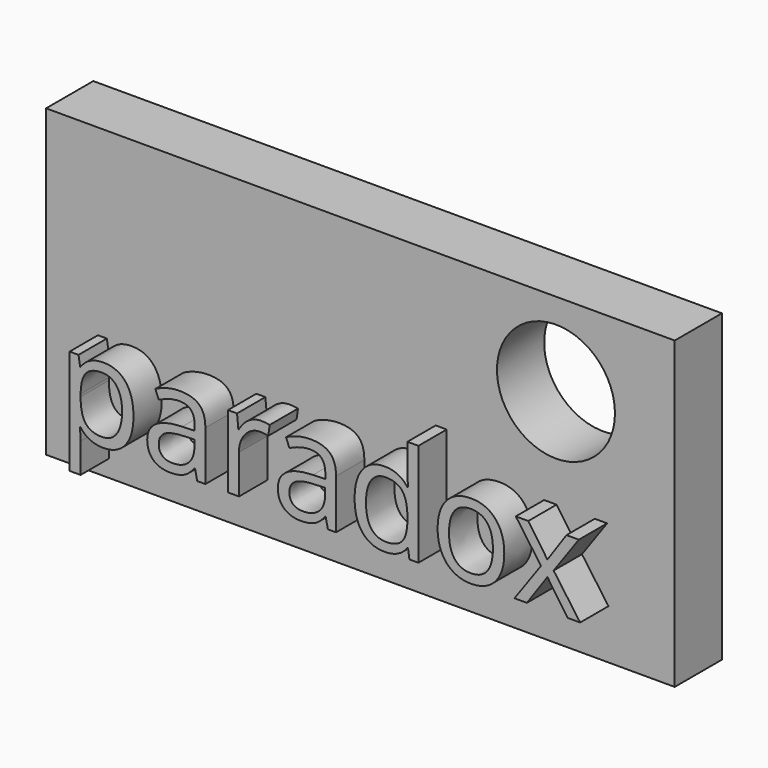
from build123d import *

# Parameters (mm, degrees)
F0_W         = 53.2775521278
F0_H         = 25.8456766605
F1_DEPTH     = 5
F2_TEXT_SIZE = 11.4827957418
F3_DEPTH     = 3
F4_R         = 5
F5_DEPTH     = 5


# Not quite as in the source:
# - Text() gives the source's letters only with a copy of the font that has no kerning and outlines rounded to 1/6400 em; it was checked with that copy


with BuildPart() as f1:
    # F0 (on Front) → F1 (new body)
    with BuildSketch(Plane.XZ):
        with Locations((26.6387760639, 12.9228383303)):
            Rectangle(F0_W, F0_H)
    extrude(amount=F1_DEPTH)

    # F2 (on face) → F3 (join)
    with BuildSketch(Plane.XZ.offset(5)):
        with Locations((3.4076778454, 4.1998989261)):
            Text('paradox', F2_TEXT_SIZE, font='Open Sans', text_align=(TextAlign.LEFT, TextAlign.BOTTOM))
    extrude(amount=F3_DEPTH)

    # F4 (on face) → F5 (cut)
    with BuildSketch(Plane.XZ.offset(5)):
        with Locations((43.2124957442, 18.762415275)):
            Circle(F4_R)
    extrude(amount=-F5_DEPTH, mode=Mode.SUBTRACT)


solid = f1.part
